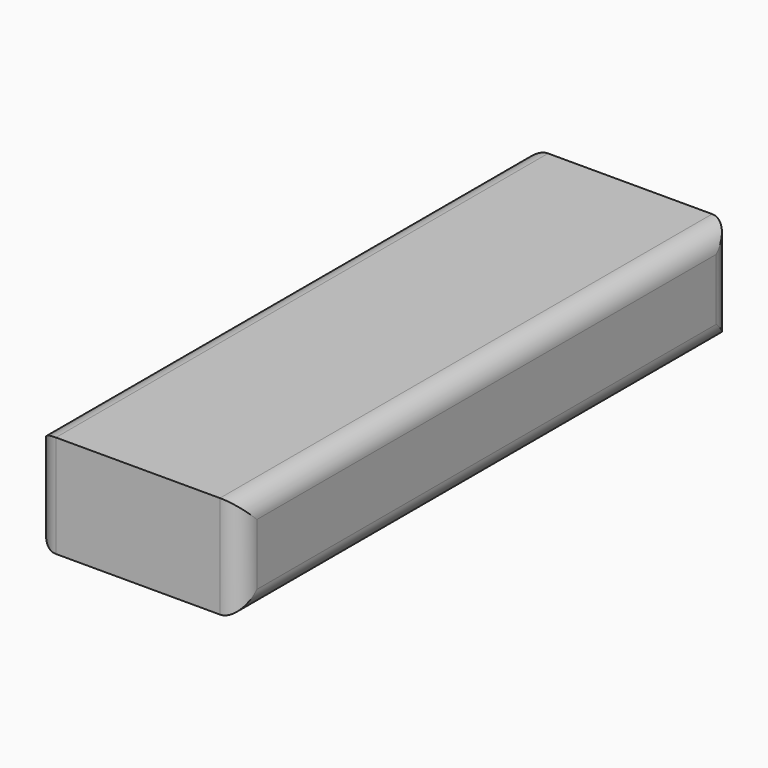
from build123d import *

# Parameters (mm, degrees)
F0_W     = 50.8
F0_H     = 152.4
F1_DEPTH = 25.4
F2_R     = 5.08
F3_T     = -2.54


# Not quite as in the source:
# - a shell that OpenCascade refuses in one call is made with other operations: the cavity is built on its own and cut out


with BuildPart() as f1:
    # F0 (on Top) → F1 (new body)
    with BuildSketch(Plane.XY):
        Rectangle(F0_W, F0_H)
    extrude(amount=F1_DEPTH)

    # F2
    f2_edges = [f1.edges().sort_by_distance(p)[0] for p in [
        (-25.4, 76.2, 12.7),
        (25.4, 76.2, 12.7),
        (-25.4, -76.2, 12.7),
        (25.4, -76.2, 12.7),
        (25.4, 0, 25.4),
        (25.4, 0, 0),
        (-25.4, 0, 25.4),
        (-25.4, 0, 0),
    ]]
    fillet(f2_edges, radius=F2_R)

    # F3: a shell. OpenCascade refuses it in one call, so the cavity is built on its own and cut out:
    # the body offset inwards by the wall thickness, plus a prism from it out through each open face.
    f3_core = offset(f1.part, amount=F3_T, mode=Mode.PRIVATE)
    f3_exits = [f3_core.faces().sort_by_distance(p)[0] for p in [
        (-22.86, 0, 12.7),
    ]]
    add(f3_core, mode=Mode.SUBTRACT)
    extrude(f3_exits, amount=-F3_T, mode=Mode.SUBTRACT)


solid = f1.part
